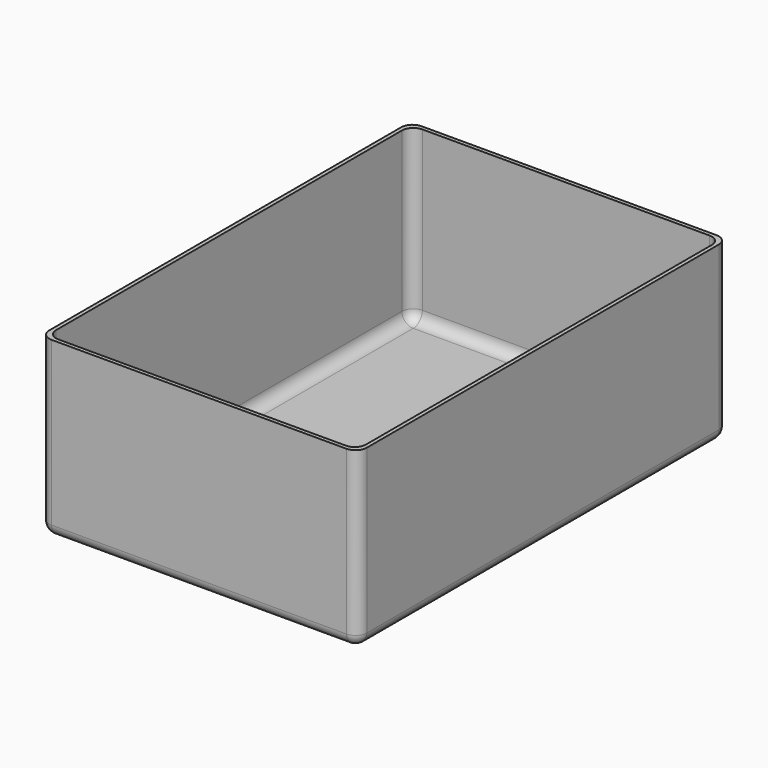
from build123d import *

# Parameters (mm, degrees)
F0_W         = 140.4
F0_H         = 204.5
F1_DEPTH     = 77.1
F2_W         = 137
F2_H         = 201.1
F3_DEPTH     = 75.4
F4_R         = 5
F5_T1_DEPTH  = 70.4
F5_S5_W      = 5
F5_S5_H      = 5
F5_T6_DEPTH  = 5
F5_S11_W     = 5
F5_S11_H     = 5
F5_T12_DEPTH = 5
F5_S17_W     = 5
F5_S17_H     = 5
F5_T18_DEPTH = 5
F5_S23_W     = 5
F5_S23_H     = 5
F5_T24_DEPTH = 5
F5_T27_DEPTH = 84.6
F5_S31_W     = 5
F5_S31_H     = 5
F5_T32_DEPTH = 5
F5_S37_W     = 5
F5_S37_H     = 5
F5_T38_DEPTH = 5
F5_S43_W     = 5
F5_S43_H     = 5
F5_T44_DEPTH = 5
F5_S49_W     = 5
F5_S49_H     = 5
F5_T50_DEPTH = 5


# Not quite as in the source:
# - a fillet or chamfer that OpenCascade refuses, or shapes differently, is made with other operations: its cross-section is extruded or revolved along the edge and cut away or added


with BuildPart() as f1:
    # F0 (on Top) → F1 (new body)
    with BuildSketch(Plane.XY):
        with Locations((70.2, 102.25)):
            Rectangle(F0_W, F0_H)
    extrude(amount=F1_DEPTH)

    # F2 (on face) → F3 (cut)
    with BuildSketch(Plane.XY.offset(77.1)):
        with Locations((70.2, 102.25)):
            Rectangle(F2_W, F2_H)
    extrude(amount=-F3_DEPTH, mode=Mode.SUBTRACT)

    # F4
    f4_edges = [f1.edges().sort_by_distance(p)[0] for p in [
        (70.2, 202.8, 1.7),
        (1.7, 102.25, 1.7),
        (70.2, 1.7, 1.7),
        (138.7, 102.25, 1.7),
        (0, 102.25, 0),
        (70.2, 0, 0),
        (140.4, 102.25, 0),
        (70.2, 204.5, 0),
    ]]
    fillet(f4_edges, radius=F4_R)

    # F5: fillet of radius 5 on 8 edges, made by hand

    # F5_s2 → F5_t1 (join)
    with BuildSketch(Plane.XY.offset(6.7)):
        with BuildLine():
            ThreePointArc((133.7, 202.8), (137.2355339059, 201.3355339059), (138.7, 197.8))
            Line((138.7, 197.8), (138.7, 202.8))
            Line((138.7, 202.8), (133.7, 202.8))
        make_face()
        with BuildLine():
            ThreePointArc((6.7, 202.8), (3.1644660941, 201.3355339059), (1.7, 197.8))
            Line((1.7, 197.8), (1.7, 202.8))
            Line((1.7, 202.8), (6.7, 202.8))
        make_face()
        with BuildLine():
            ThreePointArc((1.7, 6.7), (3.1644660941, 3.1644660941), (6.7, 1.7))
            Line((6.7, 1.7), (1.7, 1.7))
            Line((1.7, 1.7), (1.7, 6.7))
        make_face()
        with BuildLine():
            ThreePointArc((133.7, 1.7), (137.2355339059, 3.1644660941), (138.7, 6.7))
            Line((138.7, 6.7), (138.7, 1.7))
            Line((138.7, 1.7), (133.7, 1.7))
        make_face()
    extrude(amount=F5_T1_DEPTH)


with BuildPart() as f5_tool4:
    # F5_s5 → F5_t6 (new body)
    with BuildSketch(Plane.XZ.offset(-6.7)):
        with Locations((136.2, 4.2)):
            Rectangle(F5_S5_W, F5_S5_H)
    extrude(amount=F5_T6_DEPTH)

    # F5_s7 → F5_t8 (revolve, cut)
    with BuildSketch(Plane(origin=(133.7, 6.7, 6.7), x_dir=(-0.7071067812, 0, 0.7071067812), z_dir=(0.7071067812, 0, 0.7071067812))):
        with BuildLine():
            ThreePointArc((0, -5), (5, 0), (0, 5))
            Line((0, 5), (0, -5))
        make_face()
    revolve(axis=Axis((133.7, 6.7, 6.7), (0, -1, 0)), mode=Mode.SUBTRACT)


with BuildPart() as f1_1:
    add(f1.part)

    # F5_t3: union F5_tool4
    add(f5_tool4.part)


with BuildPart() as f5_tool10:
    # F5_s11 → F5_t12 (new body)
    with BuildSketch(Plane.YZ.offset(6.7)):
        with Locations((4.2, 4.2)):
            Rectangle(F5_S11_W, F5_S11_H)
    extrude(amount=-F5_T12_DEPTH)

    # F5_s13 → F5_t14 (revolve, cut)
    with BuildSketch(Plane(origin=(6.7, 6.7, 6.7), x_dir=(0, 0.7071067812, 0.7071067812), z_dir=(0, -0.7071067812, 0.7071067812))):
        with BuildLine():
            ThreePointArc((0, -5), (5, 0), (0, 5))
            Line((0, 5), (0, -5))
        make_face()
    revolve(axis=Axis((6.7, 6.7, 6.7), (-1, 0, 0)), mode=Mode.SUBTRACT)


with BuildPart() as f1_2:
    add(f1_1.part)

    # F5_t9: union F5_tool10
    add(f5_tool10.part)


with BuildPart() as f5_tool16:
    # F5_s17 → F5_t18 (new body)
    with BuildSketch(Plane.XZ.offset(-197.8)):
        with Locations((4.2, 4.2)):
            Rectangle(F5_S17_W, F5_S17_H)
    extrude(amount=-F5_T18_DEPTH)

    # F5_s19 → F5_t20 (revolve, cut)
    with BuildSketch(Plane(origin=(6.7, 197.8, 6.7), x_dir=(0.7071067812, 0, 0.7071067812), z_dir=(-0.7071067812, 0, 0.7071067812))):
        with BuildLine():
            ThreePointArc((0, -5), (5, 0), (0, 5))
            Line((0, 5), (0, -5))
        make_face()
    revolve(axis=Axis((6.7, 197.8, 6.7), (0, 1, 0)), mode=Mode.SUBTRACT)


with BuildPart() as f1_3:
    add(f1_2.part)

    # F5_t15: union F5_tool16
    add(f5_tool16.part)


with BuildPart() as f5_tool22:
    # F5_s23 → F5_t24 (new body)
    with BuildSketch(Plane.XZ.offset(-197.8)):
        with Locations((136.2, 4.2)):
            Rectangle(F5_S23_W, F5_S23_H)
    extrude(amount=-F5_T24_DEPTH)

    # F5_s25 → F5_t26 (revolve, cut)
    with BuildSketch(Plane(origin=(133.7, 197.8, 6.7), x_dir=(-0.7071067812, 0, 0.7071067812), z_dir=(-0.7071067812, 0, -0.7071067812))):
        with BuildLine():
            ThreePointArc((0, -5), (5, 0), (0, 5))
            Line((0, 5), (0, -5))
        make_face()
    revolve(axis=Axis((133.7, 197.8, 6.7), (0, 1, 0)), mode=Mode.SUBTRACT)


with BuildPart() as f1_4:
    add(f1_3.part)

    # F5_t21: union F5_tool22
    add(f5_tool22.part)

    # F5_s28 → F5_t27 (cut)
    with BuildSketch(Plane.XY.offset(5)):
        with BuildLine():
            ThreePointArc((0, 5), (1.4644660941, 1.4644660941), (5, 0))
            Line((5, 0), (0, 0))
            Line((0, 0), (0, 5))
        make_face()
        with BuildLine():
            ThreePointArc((135.4, 0), (138.9355339059, 1.4644660941), (140.4, 5))
            Line((140.4, 5), (140.4, 0))
            Line((140.4, 0), (135.4, 0))
        make_face()
        with BuildLine():
            ThreePointArc((135.4, 204.5), (138.9355339059, 203.0355339059), (140.4, 199.5))
            Line((140.4, 199.5), (140.4, 204.5))
            Line((140.4, 204.5), (135.4, 204.5))
        make_face()
        with BuildLine():
            ThreePointArc((0, 199.5), (1.4644660941, 203.0355339059), (5, 204.5))
            Line((5, 204.5), (0, 204.5))
            Line((0, 204.5), (0, 199.5))
        make_face()
    extrude(amount=F5_T27_DEPTH, mode=Mode.SUBTRACT)


with BuildPart() as f5_tool30:
    # F5_s31 → F5_t32 (new body)
    with BuildSketch(Plane.YZ.offset(5)):
        with Locations((202, 2.5)):
            Rectangle(F5_S31_W, F5_S31_H)
    extrude(amount=-F5_T32_DEPTH)

    # F5_s33 → F5_t34 (revolve, cut)
    with BuildSketch(Plane(origin=(5, 199.5, 5), x_dir=(0, -0.7071067812, 0.7071067812), z_dir=(0, -0.7071067812, -0.7071067812))):
        with BuildLine():
            ThreePointArc((0, -5), (5, 0), (0, 5))
            Line((0, 5), (0, -5))
        make_face()
    revolve(axis=Axis((5, 199.5, 5), (-1, 0, 0)), mode=Mode.SUBTRACT)


with BuildPart() as f1_5:
    add(f1_4.part)

    # F5_t29: cut F5_tool30
    add(f5_tool30.part, mode=Mode.SUBTRACT)


with BuildPart() as f5_tool36:
    # F5_s37 → F5_t38 (new body)
    with BuildSketch(Plane.XZ.offset(-199.5)):
        with Locations((137.9, 2.5)):
            Rectangle(F5_S37_W, F5_S37_H)
    extrude(amount=-F5_T38_DEPTH)

    # F5_s39 → F5_t40 (revolve, cut)
    with BuildSketch(Plane(origin=(135.4, 199.5, 5), x_dir=(-0.7071067812, 0, 0.7071067812), z_dir=(-0.7071067812, 0, -0.7071067812))):
        with BuildLine():
            ThreePointArc((0, -5), (5, 0), (0, 5))
            Line((0, 5), (0, -5))
        make_face()
    revolve(axis=Axis((135.4, 199.5, 5), (0, 1, 0)), mode=Mode.SUBTRACT)


with BuildPart() as f1_6:
    add(f1_5.part)

    # F5_t35: cut F5_tool36
    add(f5_tool36.part, mode=Mode.SUBTRACT)


with BuildPart() as f5_tool42:
    # F5_s43 → F5_t44 (new body)
    with BuildSketch(Plane.XZ.offset(-5)):
        with Locations((137.9, 2.5)):
            Rectangle(F5_S43_W, F5_S43_H)
    extrude(amount=F5_T44_DEPTH)

    # F5_s45 → F5_t46 (revolve, cut)
    with BuildSketch(Plane(origin=(135.4, 5, 5), x_dir=(-0.7071067812, 0, 0.7071067812), z_dir=(0.7071067812, 0, 0.7071067812))):
        with BuildLine():
            ThreePointArc((0, -5), (5, 0), (0, 5))
            Line((0, 5), (0, -5))
        make_face()
    revolve(axis=Axis((135.4, 5, 5), (0, -1, 0)), mode=Mode.SUBTRACT)


with BuildPart() as f1_7:
    add(f1_6.part)

    # F5_t41: cut F5_tool42
    add(f5_tool42.part, mode=Mode.SUBTRACT)


with BuildPart() as f5_tool48:
    # F5_s49 → F5_t50 (new body)
    with BuildSketch(Plane.YZ.offset(5)):
        with Locations((2.5, 2.5)):
            Rectangle(F5_S49_W, F5_S49_H)
    extrude(amount=-F5_T50_DEPTH)

    # F5_s51 → F5_t52 (revolve, cut)
    with BuildSketch(Plane(origin=(5, 5, 5), x_dir=(0, 0.7071067812, 0.7071067812), z_dir=(0, -0.7071067812, 0.7071067812))):
        with BuildLine():
            ThreePointArc((0, -5), (5, 0), (0, 5))
            Line((0, 5), (0, -5))
        make_face()
    revolve(axis=Axis((5, 5, 5), (-1, 0, 0)), mode=Mode.SUBTRACT)


with BuildPart() as f1_8:
    add(f1_7.part)

    # F5_t47: cut F5_tool48
    add(f5_tool48.part, mode=Mode.SUBTRACT)


solid = f1_8.part
